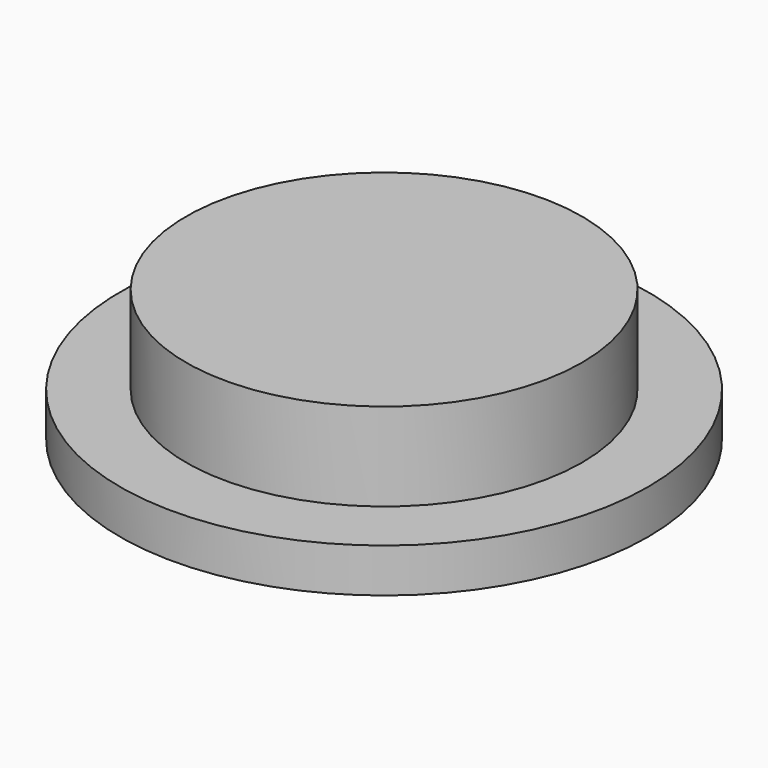
from build123d import *

# Parameters (mm, degrees)
F0_R     = 76.2
F1_DEPTH = 12.7
F6_R     = 57.15
F7_DEPTH = 38.1


# Not quite as in the source:
# - the program builds the solid bodies; features that only make, move or delete a surface that nothing else refers to are left out


with BuildPart() as f1:
    # F0 (on Top) → F1 (new body)
    with BuildSketch(Plane.XY):
        Circle(F0_R)
    extrude(amount=F1_DEPTH)

    # F6 (on Top) → F7 (join)
    with BuildSketch(Plane.XY):
        Circle(F6_R)
    extrude(amount=F7_DEPTH)


solid = f1.part
